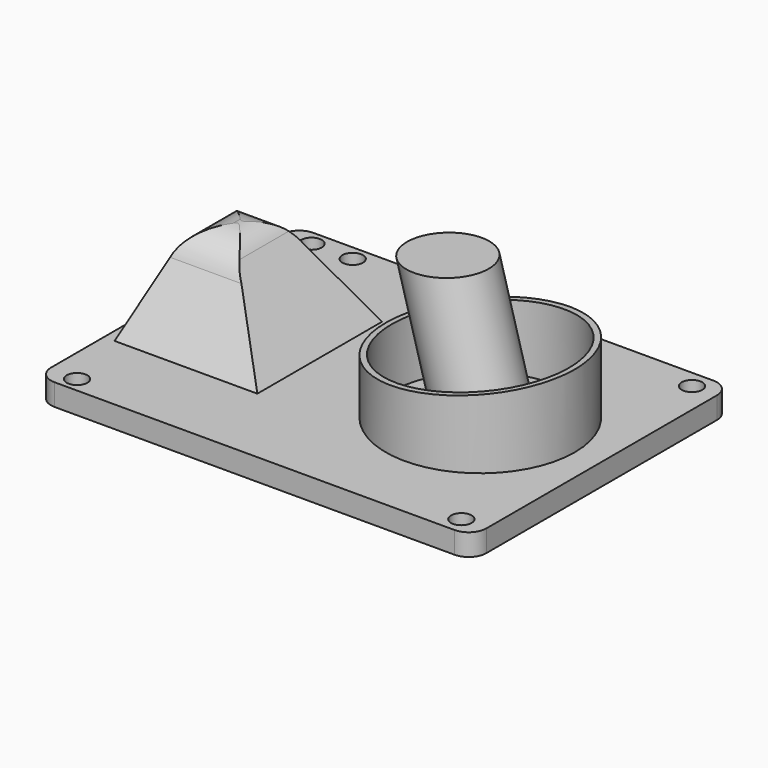
from build123d import *

# Parameters (mm, degrees)
F0_W          = 74
F0_H          = 55
F0_R          = 1.75
F0_R_2        = 16.05
F0_W_2        = 30
F0_H_2        = 26
F1_DEPTH      = 3.7
F2_DEPTH      = 16.1
F3_T          = -1
F4_R          = 3
F5_R          = 3
F6_R          = 3
F8_DEPTH      = 25
F8_DEPTH_BACK = 25
F10_DEPTH     = 13.25
F12_DEPTH     = 45
F13_T1_DEPTH  = 23.7483217569
F14_R         = 1.75
F15_DEPTH     = 104
F19_DEPTH     = 12.5


# Not quite as in the source:
# - a fillet or chamfer that OpenCascade refuses, or shapes differently, is made with other operations: its cross-section is extruded or revolved along the edge and cut away or added
# - an extrude ends at something that could not be found from the text; its depth is read off the source's solid


with BuildPart() as f1:
    # F0 (on Top) → F1 (new body)
    with BuildSketch(Plane.XY):
        Rectangle(F0_W, F0_H)
        with Locations((-32.25, -24.9075)):
            Circle(F0_R, mode=Mode.SUBTRACT)
        with Locations((32.75, -24.5)):
            Circle(F0_R, mode=Mode.SUBTRACT)
        with Locations((16.4502794727, -0.1071739239)):
            Circle(F0_R_2, mode=Mode.SUBTRACT)
        with Locations((-20.85, 0)):
            Rectangle(F0_W_2, F0_H_2, mode=Mode.SUBTRACT)
        with Locations((-32.25, 24.9075)):
            Circle(F0_R, mode=Mode.SUBTRACT)
        with Locations((-25.25, 24.9075)):
            Circle(F0_R, mode=Mode.SUBTRACT)
        with Locations((32.75, 24.5)):
            Circle(F0_R, mode=Mode.SUBTRACT)
        with Locations((16.4502794727, -0.1071739239)):
            Circle(F0_R_2)
        with Locations((-20.85, 0)):
            Rectangle(F0_W_2, F0_H_2)
    extrude(amount=F1_DEPTH)

    # F0 (on Top) → F2 (join)
    with BuildSketch(Plane.XY):
        with Locations((16.4502794727, -0.1071739239)):
            Circle(F0_R_2)
    extrude(amount=F2_DEPTH)

    # F3
    f3_openings = [f1.faces().sort_by_distance(p)[0] for p in [
        (16.450279, -0.107174, 16.1),
    ]]
    offset(amount=F3_T, openings=f3_openings, kind=Kind.INTERSECTION)

    # F4
    f4_edges = [f1.edges().sort_by_distance(p)[0] for p in [
        (37, -27.5, 1.85),
    ]]
    fillet(f4_edges, radius=F4_R)

    # F5
    f5_edges = [f1.edges().sort_by_distance(p)[0] for p in [
        (-37, -27.5, 1.85),
    ]]
    fillet(f5_edges, radius=F5_R)

    # F6
    f6_edges = [f1.edges().sort_by_distance(p)[0] for p in [
        (37, 27.5, 1.85),
        (-37, 27.5, 1.85),
    ]]
    fillet(f6_edges, radius=F6_R)

    # F7 (on Front) → F8 (cut, two sides)
    with BuildSketch(Plane.XZ) as f8_sk:
        Polygon((0.28697688, 12.6480264865), (32.789242817, 16.1480264865), (0.28697688, 16.1480264865), align=None)
    extrude(amount=-F8_DEPTH, mode=Mode.SUBTRACT)
    extrude(f8_sk.sketch, amount=F8_DEPTH_BACK, mode=Mode.SUBTRACT)

    # F9 (on Front) → F10 (join, symmetric)
    with BuildSketch(Plane.XZ):
        with BuildLine():
            Line((-35.2, 3.7), (-34, 3.7))
            Line((-34, 3.7), (-10.9234992415, 3.7))
            Line((-10.9234992415, 3.7), (-21.4788466692, 19))
            ThreePointArc((-21.4788466692, 19), (-26.9989833996, 19.0456914763), (-30.8422791347, 15.082980898))
            Line((-30.8422791347, 15.082980898), (-35.2, 3.7))
        make_face()
    extrude(amount=F10_DEPTH, both=True)

    # F11 (on Right) → F12 (cut)
    with BuildSketch(Plane.YZ):
        with BuildLine():
            ThreePointArc((-6.8658292344, 15.0277878828), (-4.1214232588, 18.344788865), (0, 19.5890275867))
            Line((0, 19.5890275867), (-13.25, 19.5890275867))
            Line((-13.25, 19.5890275867), (-13.25, 15.082980898))
            Line((-13.25, 15.082980898), (-13.25, 3.7))
            Line((-13.25, 3.7), (-6.8658292344, 15.0277878828))
        make_face()
        with BuildLine():
            Line((13.25, 3.7), (13.25, 15.082980898))
            Line((13.25, 15.082980898), (13.25, 19.5890275867))
            Line((13.25, 19.5890275867), (0, 19.5890275867))
            ThreePointArc((0, 19.5890275867), (4.1214232588, 18.344788865), (6.8658292344, 15.0277878828))
            Line((6.8658292344, 15.0277878828), (13.25, 3.7))
        make_face()
    extrude(amount=-F12_DEPTH, mode=Mode.SUBTRACT)

    # F13: fillet of radius 5 on 1 edges, made by hand

    # F13_s2 → F13_t1 (cut)
    with BuildSketch(Plane.XZ.offset(-11.8741608785)):
        with BuildLine():
            ThreePointArc((-20.3869820489, 17.4173397602), (-22.4131252415, 19.1204957059), (-25.0248198534, 19.5506673765))
            ThreePointArc((-25.0248198534, 19.5506673765), (-23.2160189055, 19.5059570206), (-21.4788466692, 19))
            Line((-21.4788466692, 19), (-20.3869820489, 17.4173397602))
        make_face()
    extrude(amount=F13_T1_DEPTH, mode=Mode.SUBTRACT)

    # F14 (on Top) → F15 (cut, through all)
    with BuildSketch(Plane.XY):
        with Locations((-32.25, 24.9075)):
            Circle(F14_R)
        with Locations((-25.25, 24.9075)):
            Circle(F14_R)
    extrude(amount=-F15_DEPTH, mode=Mode.SUBTRACT)


with BuildPart() as f17:
    # F16 (on Front) → F17 (revolve)
    with BuildSketch(Plane.XZ):
        Polygon((9.7785348499, 29.9677548091), (17.1002794727, 3.7), (24.1002794727, 3.7), (16.7785348499, 29.9677548091), align=None)
    revolve(axis=Axis((13.4394071613, 0, 16.8338774046), (-0.2684998475, 0, 0.9632797267)))

    # F18 (on Front) → F19 (cut, symmetric)
    with BuildSketch(Plane.XZ):
        Polygon((0.2809657395, 25.7425316266), (3.921539106, 25.8670715578), (17.7893069679, 26.3414723408), (18.2282145804, 32.3491258427), (4.9899508543, 32.7628237839), (2.055067569, 32.8836254776), align=None)
    extrude(amount=F19_DEPTH, both=True, mode=Mode.SUBTRACT)


solid = Compound([f1.part, f17.part])
